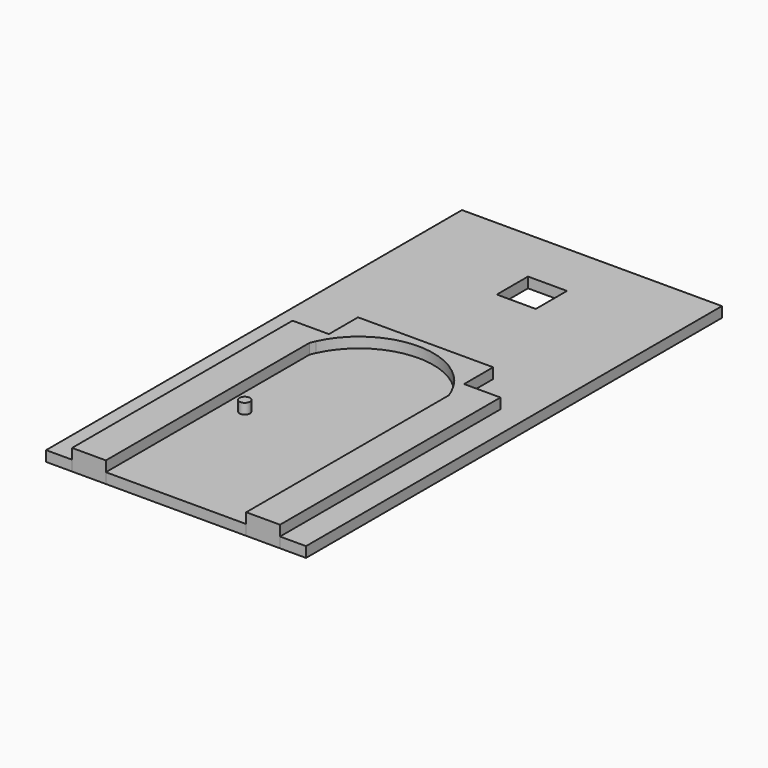
from build123d import *

# Parameters (mm, degrees)
F0_W     = 7.5
F0_H     = 7.5
F1_DEPTH = 2
F0_R     = 1
F2_DEPTH = 4


# Not quite as in the source:
# - a feature names something its author has since deleted; it is built from what else it names


with BuildPart() as f1:
    # F0 (on Top) → F1 (new body)
    with BuildSketch(Plane.XY):
        Polygon((25, -50), (25, 50), (-25, 50), (-25, -50), (-20, -50), (-20, 3), (-13, 3), (-13, 10), (-12.8840403631, 10), (13, 10), (13, 3), (20, 3), (20, -50), align=None)
        with Locations((0, 35.5613231659)):
            Rectangle(F0_W, F0_H, mode=Mode.SUBTRACT)
    extrude(amount=F1_DEPTH)


with BuildPart() as f1b:
    # F0 (on Top) → F1, piece 2 (new body)
    with BuildSketch(Plane.XY):
        with BuildLine():
            Line((-13.5, -50), (13.5, -50))
            Line((13.5, -50), (13.5, -1.2959463056))
            ThreePointArc((13.5, -1.2959463056), (13.2542929953, -0.641597419), (12.9769896425, 0))
            ThreePointArc((12.9769896425, 0), (-0.0421420295, 8.3307220269), (-13.0612737015, 0))
            ThreePointArc((-13.0612737015, 0), (-13.2912487699, -0.5257830712), (-13.5, -1.0603476549))
            Line((-13.5, -1.0603476549), (-13.5, -50))
        make_face()
        with Locations((-9.527922608, -21.5698555112)):
            Circle(F0_R, mode=Mode.SUBTRACT)
    extrude(amount=F1_DEPTH)


with BuildPart() as f2:
    # F0 (on Top) → F2 (new body)
    with BuildSketch(Plane.XY):
        with BuildLine():
            Line((13.5, -50), (20, -50))
            Line((20, -50), (20, 3))
            Line((20, 3), (13, 3))
            Line((13, 3), (13, 10))
            Line((13, 10), (-12.8840403631, 10))
            Line((-12.8840403631, 10), (-13, 10))
            Line((-13, 10), (-13, 3))
            Line((-13, 3), (-20, 3))
            Line((-20, 3), (-20, -50))
            Line((-20, -50), (-13.5, -50))
            Line((-13.5, -50), (-13.5, -1.0603476549))
            ThreePointArc((-13.5, -1.0603476549), (-13.2912487699, -0.5257830712), (-13.0612737015, 0))
            ThreePointArc((-13.0612737015, 0), (-0.0421420295, 8.3307220269), (12.9769896425, 0))
            ThreePointArc((12.9769896425, 0), (13.2542929953, -0.641597419), (13.5, -1.2959463056))
            Line((13.5, -1.2959463056), (13.5, -50))
        make_face()
    extrude(amount=F2_DEPTH)


with BuildPart() as f2b:
    # F0 (on Top) → F2, piece 2 (new body)
    with BuildSketch(Plane.XY):
        with Locations((-9.527922608, -21.5698555112)):
            Circle(F0_R)
    extrude(amount=F2_DEPTH)


solid = Compound([f1.part, f1b.part, f2.part, f2b.part])
